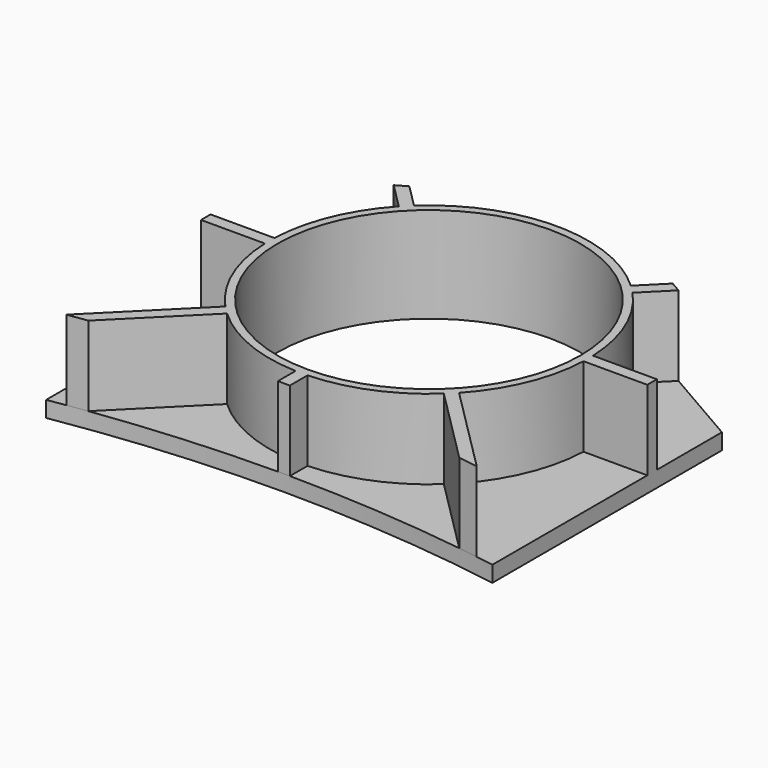
from build123d import *

# Parameters (mm, degrees)
F1_DEPTH = 25.4
F3_DEPTH = 127
F4_R     = 254
F5_DEPTH = 152.4
F6_R     = 241.3
F7_DEPTH = 152.4


with BuildPart() as f1:
    # F0 (on Top) → F1 (new body)
    with BuildSketch(Plane.XY):
        with BuildLine():
            Line((-355.6, 139.1030316258), (-355.6, -318.0850094258))
            ThreePointArc((-355.6, -318.0850094258), (0, -288.925), (355.6, -318.0850094258))
            Line((355.6, -318.0850094258), (355.6, 139.1030316258))
            Line((355.6, 139.1030316258), (101.6, 285.75))
            Line((101.6, 285.75), (-101.6, 285.75))
            Line((-101.6, 285.75), (-355.6, 139.1030316258))
        make_face()
    extrude(amount=F1_DEPTH)

    # F2 (on face) → F3 (join)
    with BuildSketch(Plane.XY.offset(25.4)):
        with BuildLine():
            Line((-209.8065405207, 223.2769247023), (-226.8863032655, 213.4159190839))
            Line((-226.8863032655, 213.4159190839), (-60.1941220043, 46.7237378227))
            ThreePointArc((-60.1941220043, 46.7237378227), (-53.8815367264, 53.8815367264), (-46.7237378227, 60.1941220043))
            Line((-46.7237378227, 60.1941220043), (-209.8065405207, 223.2769247023))
        make_face()
        with BuildLine():
            Line((-60.1941220043, -46.7237378227), (-327.0327279417, -313.5623437601))
            ThreePointArc((-327.0327279417, -313.5623437601), (-311.302932669, -311.2373508984), (-295.5566184449, -309.0270026265))
            Line((-295.5566184449, -309.0270026265), (-46.7237378227, -60.1941220043))
            ThreePointArc((-46.7237378227, -60.1941220043), (-53.8815367264, -53.8815367264), (-60.1941220043, -46.7237378227))
        make_face()
        with BuildLine():
            Line((-75.6023437137, 9.525), (-355.6, 9.525))
            Line((-355.6, 9.525), (-355.6, -9.525))
            Line((-355.6, -9.525), (-75.6023437137, -9.525))
            ThreePointArc((-75.6023437137, -9.525), (-76.2, 0), (-75.6023437137, 9.525))
        make_face()
        with BuildLine():
            Line((226.8863032655, 213.4159190839), (209.8065405207, 223.2769247023))
            Line((209.8065405207, 223.2769247023), (46.7237378227, 60.1941220043))
            ThreePointArc((46.7237378227, 60.1941220043), (53.8815367264, 53.8815367264), (60.1941220043, 46.7237378227))
            Line((60.1941220043, 46.7237378227), (226.8863032655, 213.4159190839))
        make_face()
        with BuildLine():
            Line((355.6, -9.525), (355.6, 9.525))
            Line((355.6, 9.525), (75.6023437137, 9.525))
            ThreePointArc((75.6023437137, 9.525), (76.2, 0), (75.6023437137, -9.525))
            Line((75.6023437137, -9.525), (355.6, -9.525))
        make_face()
        with BuildLine():
            Line((46.7237378227, -60.1941220043), (295.5566184449, -309.0270026265))
            ThreePointArc((295.5566184449, -309.0270026265), (311.302932669, -311.2373508984), (327.0327279417, -313.5623437601))
            Line((327.0327279417, -313.5623437601), (60.1941220043, -46.7237378227))
            ThreePointArc((60.1941220043, -46.7237378227), (53.8815367264, -53.8815367264), (46.7237378227, -60.1941220043))
        make_face()
        with BuildLine():
            Line((-9.525, -75.6023437137), (-9.525, -288.9457819171))
            Line((-9.525, -288.9457819171), (9.525, -288.9457819171))
            Line((9.525, -288.9457819171), (9.525, -75.6023437137))
            ThreePointArc((9.525, -75.6023437137), (0, -76.2), (-9.525, -75.6023437137))
        make_face()
    extrude(amount=F3_DEPTH)

    # F4 (on face) → F5 (join, through all)
    with BuildSketch(Plane(origin=(0, 0, 0), x_dir=(1, 0, 0), z_dir=(0, 0, -1))):
        Circle(F4_R)
    extrude(amount=-F5_DEPTH)

    # F6 (on face) → F7 (cut, through all)
    with BuildSketch(Plane(origin=(0, 0, 0), x_dir=(1, 0, 0), z_dir=(0, 0, -1))):
        Circle(F6_R)
    extrude(amount=-F7_DEPTH, mode=Mode.SUBTRACT)


solid = f1.part
